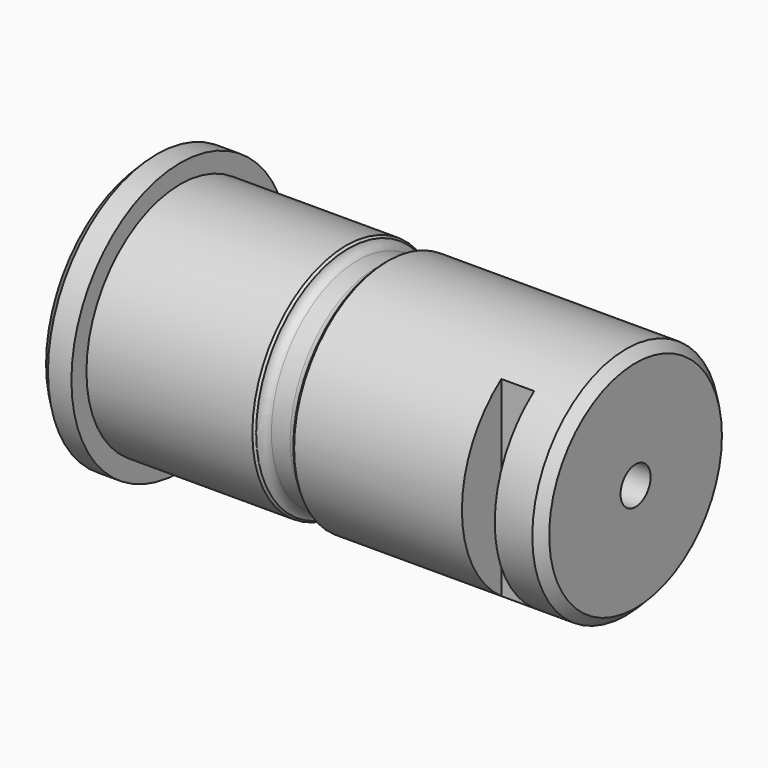
from build123d import *

# Parameters (mm, degrees)
F0_R      = 25
F1_DEPTH  = 97
F2_SIZE   = 2
F3_R      = 29
F4_DEPTH  = 7
F5_SIZE   = 2
F8_W      = 7
F8_H      = 14.5
F9_DEPTH  = 50
F11_D     = 8
F11_DEPTH = 65
F11_TIP   = 2.4034424761
F13_D     = 6
F13_DEPTH = 29.001


# Not quite as in the source:
# - a fillet or chamfer that OpenCascade refuses, or shapes differently, is made with other operations: its cross-section is extruded or revolved along the edge and cut away or added


with BuildPart() as f1:
    # F0 (on Right) → F1 (new body)
    with BuildSketch(Plane.YZ):
        Circle(F0_R)
    extrude(amount=F1_DEPTH)

    # F2
    f2_edges = [f1.edges().sort_by_distance(p)[0] for p in [
        (97, -25, 0),
    ]]
    chamfer(f2_edges, length=F2_SIZE)

    # F3 (on Right) → F4 (join)
    with BuildSketch(Plane.YZ):
        Circle(F3_R)
    extrude(amount=-F4_DEPTH)

    # F5
    f5_edges = [f1.edges().sort_by_distance(p)[0] for p in [
        (-7, -29, 0),
    ]]
    chamfer(f5_edges, length=F5_SIZE)

    # F6 (on Top) → F7 (revolve, cut)
    with BuildSketch(Plane.XY):
        with BuildLine():
            Line((43.7990407646, 27), (35.7990407646, 27))
            Line((35.7990407646, 27), (35.7990407646, 25))
            ThreePointArc((35.7990407646, 25), (36.3848272022, 23.5857864376), (37.7990407646, 23))
            Line((37.7990407646, 23), (41.7990407646, 23))
            ThreePointArc((41.7990407646, 23), (43.2132543269, 23.5857864376), (43.7990407646, 25))
            Line((43.7990407646, 25), (43.7990407646, 27))
        make_face()
    revolve(axis=Axis((58.3793800324, 0, 0), (1, 0, 0)), mode=Mode.SUBTRACT)

    # F8 (on Top) → F9 (cut, symmetric)
    with BuildSketch(Plane.XY):
        with Locations((83.5, -21.75)):
            Rectangle(F8_W, F8_H)
    extrude(amount=F9_DEPTH, both=True, mode=Mode.SUBTRACT)

    # F11
    with Locations(Plane.YZ.offset(97)):
        with Locations((0, 0)):
            Hole(F11_D / 2, depth=F11_DEPTH)
            with Locations((0, 0, -(F11_DEPTH + F11_TIP / 2))):  # 118° drill point
                Cone(0, F11_D / 2, F11_TIP, mode=Mode.SUBTRACT)

    # F13 (through all, one way)
    with BuildSketch(Plane.XY):
        with Locations((39.7990407646, 0)):
            Circle(F13_D / 2)
    extrude(amount=-F13_DEPTH, mode=Mode.SUBTRACT)

    # F14: chamfer of 0.5 on 2 edges, made by hand

    # F14_s1 → F14_t2 (revolve, cut)
    with BuildSketch(Plane.XY):
        with BuildLine():
            Line((35.3495510218, 25), (35.8394489703, 24.6))
            ThreePointArc((35.8394489703, 24.6), (35.8098979776, 24.7918871147), (35.7990407646, 25))
            Line((35.7990407646, 25), (35.3495510218, 25))
        make_face()
    revolve(axis=Axis((35.7990407646, 0, 0), (1, 0, 0)), mode=Mode.SUBTRACT)

    # F14_s3 → F14_t4 (revolve, cut)
    with BuildSketch(Plane.XY):
        with BuildLine():
            Line((43.7586325588, 24.6), (44.2485305074, 25))
            Line((44.2485305074, 25), (43.7990407646, 25))
            ThreePointArc((43.7990407646, 25), (43.7881835515, 24.7918871147), (43.7586325588, 24.6))
        make_face()
    revolve(axis=Axis((43.7990407646, 0, 0), (1, 0, 0)), mode=Mode.SUBTRACT)


solid = f1.part
